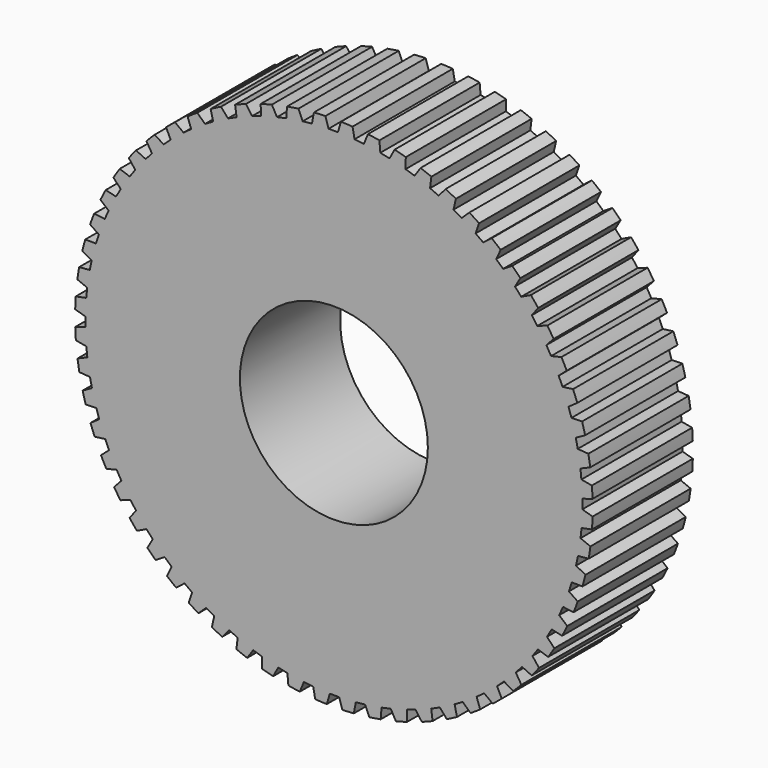
from build123d import *

# Parameters (mm, degrees)
F0_R            = 52.451
F0_R_2          = 19.05
F1_DEPTH        = 25.4
F3_DEPTH        = 25.4
F3_COPIES_COUNT = 60


# Not quite as in the source:
# - a pattern or mirror of a feature is missing from the dataset's text; its kind, count and spacing are read off the source's solid
# - a feature names something its author has since deleted; it is built from what else it names


with BuildPart() as f1:
    # F0 (on Front) → F1 (new body)
    with BuildSketch(Plane.XZ):
        Circle(F0_R)
        Circle(F0_R_2, mode=Mode.SUBTRACT)
    extrude(amount=F1_DEPTH)

    # F2 (on face) → F3 (cut)
    with BuildSketch(Plane(origin=(0, 0, 0), x_dir=(-1, 0, 0), z_dir=(0, 1, 0))):
        with BuildLine():
            ThreePointArc((1.7097625282, 52.4231257471), (0.1365637198, 52.4508222181), (-1.4367579823, 52.4313181934))
            Line((-1.4367579823, 52.4313181934), (-0.8296424614, 50.3594369844))
            Line((-0.8296424614, 50.3594369844), (1.0753575386, 50.3594369844))
            Line((1.0753575386, 50.3594369844), (1.7097625282, 52.4231257471))
        make_face()
    f3 = extrude(amount=-F3_DEPTH, mode=Mode.SUBTRACT)

    # F3_copies: F3 ×60 about axis
    f3_copies_axis = Axis((0, 0, 0), (0, 1, 0))
    for i in range(1, F3_COPIES_COUNT):
        add(f3.rotate(f3_copies_axis, i * 360 / F3_COPIES_COUNT), mode=Mode.SUBTRACT)


solid = f1.part
